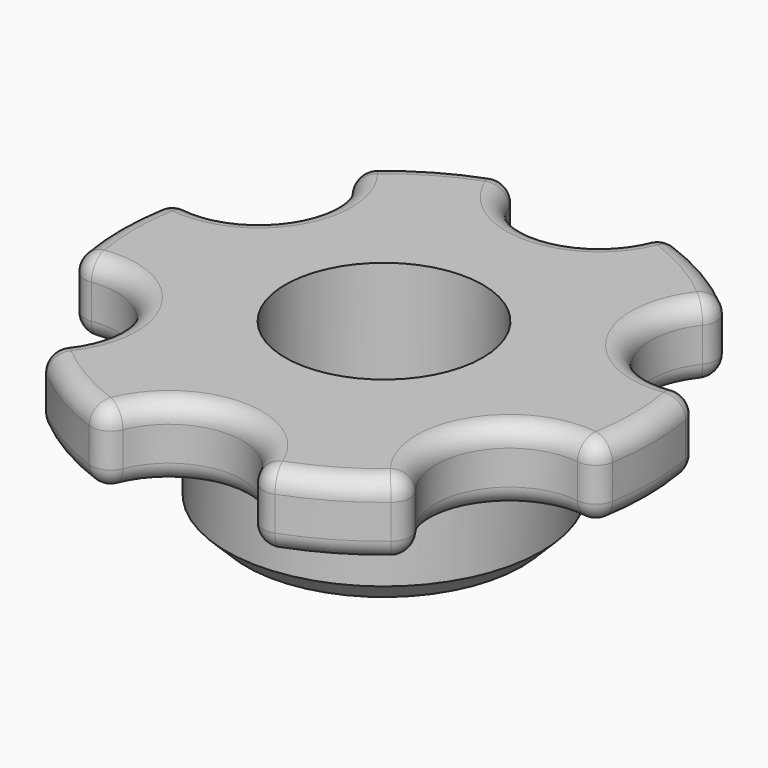
from build123d import *

# Parameters (mm, degrees)
F2_SIZE         = 2.54
F3_R            = 9.525
F4_DEPTH        = 22.226
F4_COPIES_COUNT = 6
F6_R            = 2.54


# Not quite as in the source:
# - a feature of the source that left no trace in its solid (it failed there, or was rolled back) is left out
# - a pattern or mirror of a feature is missing from the dataset's text; its kind, count and spacing are read off the source's solid


with BuildPart() as f1:
    # F0 (on Front) → F1 (revolve)
    with BuildSketch(Plane.XZ):
        Polygon((12.827, 22.225), (12.827, 0), (20.447, 0), (20.447, 12.7), (34.925, 12.7), (34.925, 22.225), align=None)
    revolve(axis=Axis((0, 0, 15.6002613144), (0, 0, 1)))

    # F2
    f2_edges = [f1.edges().sort_by_distance(p)[0] for p in [
        (-20.447, 0, 0),
    ]]
    chamfer(f2_edges, length=F2_SIZE)

    # F3 (on face) → F4 (cut, through all)
    with BuildSketch(Plane.XY.offset(22.225)):
        with Locations((0, 34.925)):
            Circle(F3_R)
    f4 = extrude(amount=-F4_DEPTH, mode=Mode.SUBTRACT)

    # F4_copies: F4 ×6 about axis
    f4_copies_axis = Axis((0, 0, 0), (0, 0, 1))
    for i in range(1, F4_COPIES_COUNT):
        add(f4.rotate(f4_copies_axis, i * 360 / F4_COPIES_COUNT), mode=Mode.SUBTRACT)

    # F6
    f6_edges = [f1.edges().sort_by_distance(p)[0] for p in [
        (0, 25.4, 22.225),
        (17.4625, 30.245937, 22.225),
        (21.997045, 12.7, 22.225),
        (34.925, 0, 22.225),
        (21.997045, -12.7, 22.225),
        (17.4625, -30.245937, 22.225),
        (0, -25.4, 22.225),
        (-17.4625, -30.245937, 22.225),
        (-21.997045, -12.7, 22.225),
        (-34.925, 0, 22.225),
        (-21.997045, 12.7, 22.225),
        (-17.4625, 30.245937, 22.225),
        (-21.997045, -12.7, 12.7),
        (-17.4625, -30.245937, 12.7),
        (0, -25.4, 12.7),
        (17.4625, -30.245937, 12.7),
        (21.997045, -12.7, 12.7),
        (34.925, 0, 12.7),
        (21.997045, 12.7, 12.7),
        (17.4625, 30.245937, 12.7),
        (0, 25.4, 12.7),
        (-17.4625, 30.245937, 12.7),
        (-21.997045, 12.7, 12.7),
        (-34.925, 0, 12.7),
        (9.436026, 33.626136, 17.4625),
        (-9.436026, 33.626136, 17.4625),
        (24.403076, 24.984906, 17.4625),
        (33.839101, 8.64123, 17.4625),
        (33.839101, -8.64123, 17.4625),
        (24.403076, -24.984906, 17.4625),
        (9.436026, -33.626136, 17.4625),
        (-9.436026, -33.626136, 17.4625),
        (-24.403076, -24.984906, 17.4625),
        (-33.839101, -8.64123, 17.4625),
        (-33.839101, 8.64123, 17.4625),
        (-24.403076, 24.984906, 17.4625),
    ]]
    fillet(f6_edges, radius=F6_R)


solid = f1.part
